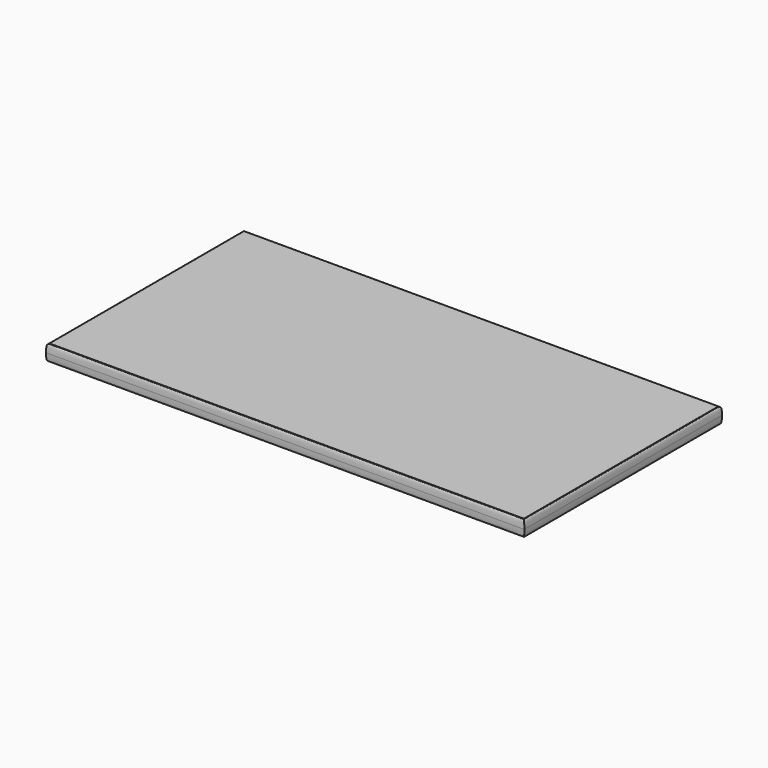
from build123d import *

# Parameters (mm, degrees)
F0_W     = 1200
F0_H     = 620
F1_DEPTH = 40
F3_DEPTH = 620.001
F6_DEPTH = 1200.0010001015


# Not quite as in the source:
# - ends of sketch curves that miss each other by under 0.0002 mm in the source are joined


with BuildPart() as f1:
    # F0 (on Top) → F1 (new body)
    with BuildSketch(Plane.XY):
        with Locations((600, 310)):
            Rectangle(F0_W, F0_H)
    extrude(amount=F1_DEPTH)

    # F2 (on face) → F3 (cut, through all)
    with BuildSketch(Plane.XZ):
        with BuildLine():
            add(Edge.make_bspline(
                [(4, 1), (0, 1), (0, 8.5583151877), (0, 20)],
                knots=[0, 0, 0, 0, 19.4164878389, 19.4164878389, 19.4164878389, 19.4164878389], degree=3))
            Line((0, 20), (0, 0))
            Line((0, 0), (5, 0))
            Line((5, 0), (5, 1))
            Line((5, 1), (4, 1))
        make_face()
        with BuildLine():
            add(Edge.make_bspline(
                [(4, 39), (0, 39), (0, 31.4416848123), (0, 20)],
                knots=[0, 0, 0, 0, 19.4164878389, 19.4164878389, 19.4164878389, 19.4164878389], degree=3))
            Line((4, 39), (5, 39))
            Line((5, 39), (5, 40))
            Line((5, 40), (0, 40))
            Line((0, 40), (0, 20))
        make_face()
        with BuildLine():
            add(Edge.make_bspline(
                [(1196, 39), (1200, 39), (1200, 31.4416848123), (1200, 20)],
                knots=[0, 0, 0, 0, 19.4164878389, 19.4164878389, 19.4164878389, 19.4164878389], degree=3))
            Line((1200, 20), (1200, 40))
            Line((1200, 40), (1195, 40))
            Line((1195, 40), (1195, 39))
            Line((1195, 39), (1196, 39))
        make_face()
        with BuildLine():
            Line((1195, 1), (1195, 0))
            Line((1195, 0), (1200, 0))
            Line((1200, 0), (1200, 20))
            add(Edge.make_bspline(
                [(1196, 1), (1200, 1), (1200, 8.5583151877), (1200, 20)],
                knots=[0, 0, 0, 0, 19.4164878389, 19.4164878389, 19.4164878389, 19.4164878389], degree=3))
            Line((1196, 1), (1195, 1))
        make_face()
    extrude(amount=-F3_DEPTH, mode=Mode.SUBTRACT)

    # F5 (on offset) → F6 (cut, through all)
    with BuildSketch(Plane(origin=(0, 0, 0), x_dir=(0, -1, 0), z_dir=(-1, 0, 0))):
        with BuildLine():
            add(Edge.make_bspline(
                [(-616.000000023, 1), (-620, 1), (-620, 8.5583149148), (-620, 19.9999997259)],
                knots=[0, 0, 0, 0, 19.416487566, 19.416487566, 19.416487566, 19.416487566], degree=3))
            Line((-620, 19.9999997259), (-620, 0))
            Line((-620, 0), (-615, 0))
            Line((-615, 0), (-615, 1))
            Line((-615, 1), (-616.000000023, 1))
        make_face()
        with BuildLine():
            add(Edge.make_bspline(
                [(-616.000000023, 39), (-620, 39), (-620, 31.4416850852), (-620, 20.0000002741)],
                knots=[0, 0, 0, 0, 19.416487566, 19.416487566, 19.416487566, 19.416487566], degree=3))
            Line((-616.000000023, 39), (-615, 39))
            Line((-615, 39), (-615, 40))
            Line((-615, 40), (-620, 40))
            Line((-620, 40), (-620, 20.0000002741))
        make_face()
        with BuildLine():
            add(Edge.make_bspline(
                [(-3.999999977, 39), (0, 39), (0, 31.4416850853), (0, 20.0000002741)],
                knots=[0, 0, 0, 0, 19.416487566, 19.416487566, 19.416487566, 19.416487566], degree=3))
            Line((0, 20.0000002741), (0, 40))
            Line((0, 40), (-5, 40))
            Line((-5, 40), (-5, 39))
            Line((-5, 39), (-3.999999977, 39))
        make_face()
        with BuildLine():
            Line((-5, 1), (-5, 0))
            Line((-5, 0), (0, 0))
            Line((0, 0), (0, 20))
            add(Edge.make_bspline(
                [(-3.999999977, 1), (0, 1), (0, 8.5583149148), (0, 20)],
                knots=[0, 0, 0, 0, 19.416487566, 19.416487566, 19.416487566, 19.416487566], degree=3))
            Line((-3.999999977, 1), (-5, 1))
        make_face()
    extrude(amount=-F6_DEPTH, mode=Mode.SUBTRACT)


solid = f1.part
